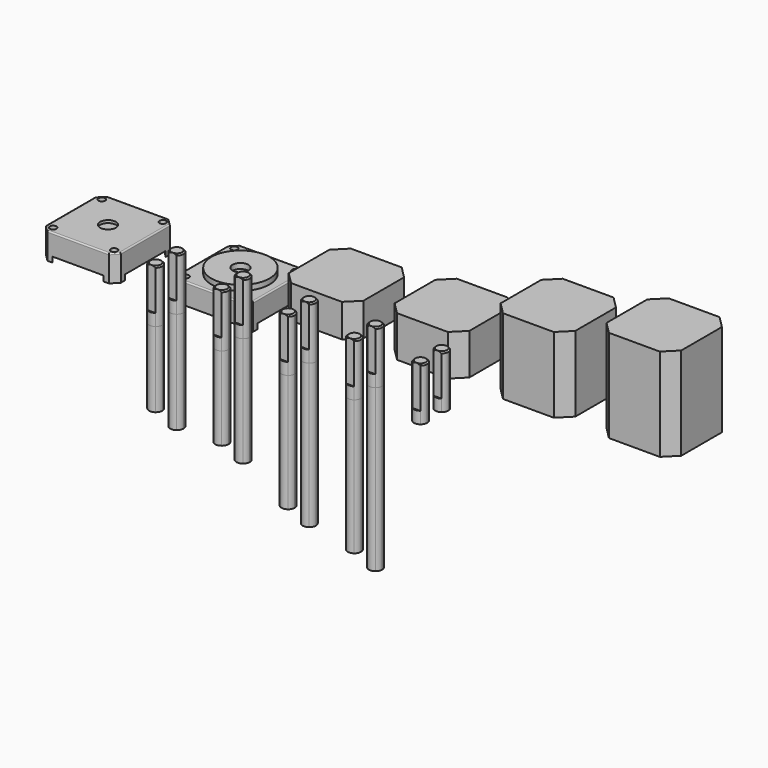
from build123d import *

# Parameters (mm, degrees)
F0_R        = 3
F1_DEPTH    = 8
F0_R_2      = 11
F2_DEPTH    = 2
F3_DEPTH    = 1
F5_DEPTH    = 2
F6_D        = 2.5
F6_DEPTH    = 3
F6_TIP      = 0.7510757738
F6_2_D      = 2.5
F6_2_DEPTH  = 3
F6_2_TIP    = 0.7510757738
F7_DEPTH    = 12.5
F8_DEPTH    = 15.5
F9_DEPTH    = 28.5
F10_DEPTH   = 35
F11_DEPTH   = 20
F13_DEPTH   = 15.5
F14_R       = 0.5
F14_2_R     = 0.5
F15_SIZE    = 0.49999
F15_2_SIZE  = 0.49999
F15_3_SIZE  = 0.49999
F15_4_SIZE  = 0.49999
F15_5_SIZE  = 0.49999
F15_6_SIZE  = 0.49999
F15_7_SIZE  = 0.49999
F15_8_SIZE  = 0.49999
F15_9_SIZE  = 0.49999
F15_10_SIZE = 0.49999
F16_DEPTH   = 28.5
F17_DEPTH   = 38.5
F18_DEPTH   = 31.5
F19_DEPTH   = 41.5
F20_DEPTH   = 44.5
F21_DEPTH   = 54.5
F22_DEPTH   = 51
F23_DEPTH   = 61


# Not quite as in the source:
# - a fillet or chamfer is up to 0.001 mm smaller than in the source, because OpenCascade refuses the exact size
# - a feature names something its author has since deleted; it is built from what else it names


with BuildPart() as f1:
    # F0 (on Top) → F1 (new body)
    with BuildSketch(Plane.XY):
        Polygon((-64.1, 9.6), (-64.1, -9.6), (-59.6, -14.1), (-40.4, -14.1), (-35.9, -9.6), (-35.9, 9.6), (-40.4, 14.1), (-59.6, 14.1), align=None)
        with Locations((-50, 0)):
            Circle(F0_R, mode=Mode.SUBTRACT)
        Polygon((-38.4, 14.1), (-40.4, 14.1), (-35.9, 9.6), (-35.9, 11.6), align=None)
        Polygon((-64.1, 11.6), (-64.1, 9.6), (-59.6, 14.1), (-61.6, 14.1), align=None)
        Polygon((-64.1, -9.6), (-64.1, -11.6), (-61.6, -14.1), (-59.6, -14.1), align=None)
        Polygon((-35.9, -9.6), (-40.4, -14.1), (-38.4, -14.1), (-35.9, -11.6), align=None)
        with Locations((-50, 0)):
            Circle(F0_R)
    extrude(amount=-F1_DEPTH)

    # F0 (on Top) → F3 (cut)
    with BuildSketch(Plane.XY):
        with Locations((-50, 0)):
            Circle(F0_R)
    extrude(amount=-F3_DEPTH, mode=Mode.SUBTRACT)

    # F4 (on face) → F5 (join)
    with BuildSketch(Plane(origin=(0, 0, -8), x_dir=(1, 0, 0), z_dir=(0, 0, -1))):
        Polygon((-35.9, -9.6), (-40.4, -14.1), (-38.4, -14.1), (-35.9, -11.6), align=None)
        Polygon((-61.6, -14.1), (-59.6, -14.1), (-64.1, -9.6), (-64.1, -11.6), align=None)
        Polygon((-64.1, 9.6), (-59.6, 14.1), (-61.6, 14.1), (-64.1, 11.6), align=None)
        Polygon((-35.9, 9.6), (-35.9, 11.6), (-38.4, 14.1), (-40.4, 14.1), align=None)
    extrude(amount=F5_DEPTH)

    # F6
    with Locations(Plane.XY):
        with Locations((-11.5, -11.5), (11.5, -11.5), (11.5, 11.5), (-11.5, 11.5), (-38.5, -11.5), (-38.5, 11.5), (-61.5, 11.5), (-61.5, -11.5)):
            Hole(F6_D / 2, depth=F6_DEPTH)
            with Locations((0, 0, -(F6_DEPTH + F6_TIP / 2))):  # 118° drill point
                Cone(0, F6_D / 2, F6_TIP, mode=Mode.SUBTRACT)

    # F14
    f14_edges = [f1.edges().sort_by_distance(p)[0] for p in [
        (-35.9, 0, 0),
        (-37.15, -12.85, 0),
        (-62.85, -12.85, 0),
        (-64.1, 0, 0),
        (-50, -14.1, 0),
        (-50, 14.1, 0),
        (-37.15, 12.85, 0),
        (-62.85, 12.85, 0),
    ]]
    fillet(f14_edges, radius=F14_R)


with BuildPart() as f1b:
    # F0 (on Top) → F1, piece 2 (new body)
    with BuildSketch(Plane.XY):
        Polygon((-9.6, -14.1), (9.6, -14.1), (14.1, -9.6), (14.1, 9.6), (9.6, 14.1), (-9.6, 14.1), (-14.1, 9.6), (-14.1, -9.6), align=None)
        Circle(F0_R_2, mode=Mode.SUBTRACT)
        Circle(F0_R_2)
        Circle(F0_R, mode=Mode.SUBTRACT)
        Polygon((-11.6, -14.1), (-9.6, -14.1), (-14.1, -9.6), (-14.1, -11.6), align=None)
        Polygon((-14.1, 11.6), (-14.1, 9.6), (-9.6, 14.1), (-11.6, 14.1), align=None)
        Polygon((9.6, 14.1), (14.1, 9.6), (14.1, 11.6), (11.6, 14.1), align=None)
        Polygon((9.6, -14.1), (11.6, -14.1), (14.1, -11.6), (14.1, -9.6), align=None)
        Circle(F0_R)
    extrude(amount=-F1_DEPTH)

    # F0 (on Top) → F2 (join)
    with BuildSketch(Plane.XY):
        Circle(F0_R_2)
        Circle(F0_R, mode=Mode.SUBTRACT)
    extrude(amount=F2_DEPTH)

    # F4 (on face) → F5, piece 2 (join)
    with BuildSketch(Plane(origin=(0, 0, -8), x_dir=(1, 0, 0), z_dir=(0, 0, -1))):
        Polygon((-11.6, -14.1), (-9.6, -14.1), (-14.1, -9.6), (-14.1, -11.6), align=None)
        Polygon((14.1, -9.6), (9.6, -14.1), (11.6, -14.1), (14.1, -11.6), align=None)
        Polygon((9.6, 14.1), (14.1, 9.6), (14.1, 11.6), (11.6, 14.1), align=None)
        Polygon((-14.1, 11.6), (-14.1, 9.6), (-9.6, 14.1), (-11.6, 14.1), align=None)
    extrude(amount=F5_DEPTH)

    # F6#2
    with Locations(Plane.XY):
        with Locations((-11.5, -11.5), (11.5, -11.5), (11.5, 11.5), (-11.5, 11.5), (-38.5, -11.5), (-38.5, 11.5), (-61.5, 11.5), (-61.5, -11.5)):
            Hole(F6_2_D / 2, depth=F6_2_DEPTH)
            with Locations((0, 0, -(F6_2_DEPTH + F6_2_TIP / 2))):  # 118° drill point
                Cone(0, F6_2_D / 2, F6_2_TIP, mode=Mode.SUBTRACT)

    # F14#2
    f14_2_edges = [f1b.edges().sort_by_distance(p)[0] for p in [
        (-14.1, 0, 0),
        (-12.85, -12.85, 0),
        (0, -14.1, 0),
        (12.85, -12.85, 0),
        (14.1, 0, 0),
        (12.85, 12.85, 0),
        (0, 14.1, 0),
        (-12.85, 12.85, 0),
    ]]
    fillet(f14_2_edges, radius=F14_2_R)


with BuildPart() as f7:
    # F0 (on Top) → F7 (new body)
    with BuildSketch(Plane.XY):
        Polygon((30.4, -14.1), (49.6, -14.1), (54.1, -9.6), (54.1, 9.6), (49.6, 14.1), (30.4, 14.1), (25.9, 9.6), (25.9, -9.6), align=None)
    extrude(amount=F7_DEPTH)


with BuildPart() as f8:
    # F0 (on Top) → F8 (new body)
    with BuildSketch(Plane.XY):
        Polygon((70.4, -14.1), (89.6, -14.1), (94.1, -9.6), (94.1, 9.6), (89.6, 14.1), (70.4, 14.1), (65.9, 9.6), (65.9, -9.6), align=None)
    extrude(amount=F8_DEPTH)


with BuildPart() as f9:
    # F0 (on Top) → F9 (new body)
    with BuildSketch(Plane.XY):
        Polygon((110.4, -14.1), (129.6, -14.1), (134.1, -9.6), (134.1, 9.6), (129.6, 14.1), (110.4, 14.1), (105.9, 9.6), (105.9, -9.6), align=None)
    extrude(amount=F9_DEPTH)


with BuildPart() as f10:
    # F0 (on Top) → F10 (new body)
    with BuildSketch(Plane.XY):
        Polygon((150.4, -14.1), (169.6, -14.1), (174.1, -9.6), (174.1, 9.6), (169.6, 14.1), (150.4, 14.1), (145.9, 9.6), (145.9, -9.6), align=None)
    extrude(amount=F10_DEPTH)


with BuildPart() as f11:
    # F0 (on Top) → F11 (new body)
    with BuildSketch(Plane.XY):
        with BuildLine():
            Line((1.5, -42), (-1.5, -42))
            ThreePointArc((-1.5, -42), (0, -42.5), (1.5, -42))
        make_face()
        with BuildLine():
            ThreePointArc((1.5, -42), (2.2360679775, -41.1180339887), (2.5, -40))
            ThreePointArc((2.5, -40), (-1.1180339887, -37.7639320225), (-1.5, -42))
            Line((-1.5, -42), (1.5, -42))
        make_face()
    extrude(amount=F11_DEPTH)


with BuildPart() as f11b:
    # F0 (on Top) → F11, piece 2 (new body)
    with BuildSketch(Plane.XY):
        with BuildLine():
            Line((1.5, -32), (-1.5, -32))
            ThreePointArc((-1.5, -32), (0, -32.5), (1.5, -32))
        make_face()
        with BuildLine():
            ThreePointArc((1.5, -32), (2.2360679775, -31.1180339887), (2.5, -30))
            ThreePointArc((2.5, -30), (-1.1180339887, -27.7639320225), (-1.5, -32))
            Line((-1.5, -32), (1.5, -32))
        make_face()
    extrude(amount=F11_DEPTH)


with BuildPart() as f11c:
    # F0 (on Top) → F11, piece 3 (new body)
    with BuildSketch(Plane.XY):
        with BuildLine():
            ThreePointArc((26.5, -42), (27.2360679775, -41.1180339887), (27.5, -40))
            ThreePointArc((27.5, -40), (23.8819660113, -37.7639320225), (23.5, -42))
            Line((23.5, -42), (26.5, -42))
        make_face()
        with BuildLine():
            Line((26.5, -42), (23.5, -42))
            ThreePointArc((23.5, -42), (25, -42.5), (26.5, -42))
        make_face()
    extrude(amount=F11_DEPTH)


with BuildPart() as f11d:
    # F0 (on Top) → F11, piece 4 (new body)
    with BuildSketch(Plane.XY):
        with BuildLine():
            ThreePointArc((26.5, -32), (27.2360679775, -31.1180339887), (27.5, -30))
            ThreePointArc((27.5, -30), (23.8819660113, -27.7639320225), (23.5, -32))
            Line((23.5, -32), (26.5, -32))
        make_face()
        with BuildLine():
            Line((26.5, -32), (23.5, -32))
            ThreePointArc((23.5, -32), (25, -32.5), (26.5, -32))
        make_face()
    extrude(amount=F11_DEPTH)


with BuildPart() as f11e:
    # F0 (on Top) → F11, piece 5 (new body)
    with BuildSketch(Plane.XY):
        with BuildLine():
            ThreePointArc((51.5, -32), (52.2360679775, -31.1180339887), (52.5, -30))
            ThreePointArc((52.5, -30), (48.8819660113, -27.7639320225), (48.5, -32))
            Line((48.5, -32), (51.5, -32))
        make_face()
        with BuildLine():
            Line((51.5, -32), (48.5, -32))
            ThreePointArc((48.5, -32), (50, -32.5), (51.5, -32))
        make_face()
    extrude(amount=F11_DEPTH)


with BuildPart() as f11f:
    # F0 (on Top) → F11, piece 6 (new body)
    with BuildSketch(Plane.XY):
        with BuildLine():
            ThreePointArc((51.5, -42), (52.2360679775, -41.1180339887), (52.5, -40))
            ThreePointArc((52.5, -40), (48.8819660113, -37.7639320225), (48.5, -42))
            Line((48.5, -42), (51.5, -42))
        make_face()
        with BuildLine():
            Line((51.5, -42), (48.5, -42))
            ThreePointArc((48.5, -42), (50, -42.5), (51.5, -42))
        make_face()
    extrude(amount=F11_DEPTH)


with BuildPart() as f11g:
    # F0 (on Top) → F11, piece 7 (new body)
    with BuildSketch(Plane.XY):
        with BuildLine():
            Line((101.5, -32), (98.5, -32))
            ThreePointArc((98.5, -32), (100, -32.5), (101.5, -32))
        make_face()
        with BuildLine():
            ThreePointArc((101.5, -32), (102.2360679775, -31.1180339887), (102.5, -30))
            ThreePointArc((102.5, -30), (98.8819660113, -27.7639320225), (98.5, -32))
            Line((98.5, -32), (101.5, -32))
        make_face()
    extrude(amount=F11_DEPTH)


with BuildPart() as f11h:
    # F0 (on Top) → F11, piece 8 (new body)
    with BuildSketch(Plane.XY):
        with BuildLine():
            ThreePointArc((101.5, -42), (102.2360679775, -41.1180339887), (102.5, -40))
            ThreePointArc((102.5, -40), (98.8819660113, -37.7639320225), (98.5, -42))
            Line((98.5, -42), (101.5, -42))
        make_face()
        with BuildLine():
            Line((101.5, -42), (98.5, -42))
            ThreePointArc((98.5, -42), (100, -42.5), (101.5, -42))
        make_face()
    extrude(amount=F11_DEPTH)


with BuildPart() as f11i:
    # F0 (on Top) → F11, piece 9 (new body)
    with BuildSketch(Plane.XY):
        with BuildLine():
            ThreePointArc((76.5, -32), (77.2360679775, -31.1180339887), (77.5, -30))
            ThreePointArc((77.5, -30), (73.8819660113, -27.7639320225), (73.5, -32))
            Line((73.5, -32), (76.5, -32))
        make_face()
        with BuildLine():
            Line((76.5, -32), (73.5, -32))
            ThreePointArc((73.5, -32), (75, -32.5), (76.5, -32))
        make_face()
    extrude(amount=F11_DEPTH)


with BuildPart() as f11j:
    # F0 (on Top) → F11, piece 10 (new body)
    with BuildSketch(Plane.XY):
        with BuildLine():
            ThreePointArc((76.5, -42), (77.2360679775, -41.1180339887), (77.5, -40))
            ThreePointArc((77.5, -40), (73.8819660113, -37.7639320225), (73.5, -42))
            Line((73.5, -42), (76.5, -42))
        make_face()
        with BuildLine():
            Line((76.5, -42), (73.5, -42))
            ThreePointArc((73.5, -42), (75, -42.5), (76.5, -42))
        make_face()
    extrude(amount=F11_DEPTH)


with BuildPart() as f13_tool:
    # F12 (on face) → F13 (new body)
    with BuildSketch(Plane.XY.offset(20)):
        with BuildLine():
            ThreePointArc((98.5, -32), (100, -32.5), (101.5, -32))
            Line((101.5, -32), (98.5, -32))
        make_face()
        with BuildLine():
            ThreePointArc((98.5, -42), (100, -42.5), (101.5, -42))
            Line((101.5, -42), (98.5, -42))
        make_face()
        with BuildLine():
            ThreePointArc((73.5, -42), (75, -42.5), (76.5, -42))
            Line((76.5, -42), (73.5, -42))
        make_face()
        with BuildLine():
            ThreePointArc((73.5, -32), (75, -32.5), (76.5, -32))
            Line((76.5, -32), (73.5, -32))
        make_face()
        with BuildLine():
            ThreePointArc((48.5, -32), (50, -32.5), (51.5, -32))
            Line((51.5, -32), (48.5, -32))
        make_face()
        with BuildLine():
            ThreePointArc((48.5, -42), (50, -42.5), (51.5, -42))
            Line((51.5, -42), (48.5, -42))
        make_face()
        with BuildLine():
            ThreePointArc((23.5, -32), (25, -32.5), (26.5, -32))
            Line((26.5, -32), (23.5, -32))
        make_face()
        with BuildLine():
            ThreePointArc((23.5, -42), (25, -42.5), (26.5, -42))
            Line((26.5, -42), (23.5, -42))
        make_face()
        with BuildLine():
            ThreePointArc((-1.5, -32), (0, -32.5), (1.5, -32))
            Line((1.5, -32), (-1.5, -32))
        make_face()
        with BuildLine():
            ThreePointArc((-1.5, -42), (0, -42.5), (1.5, -42))
            Line((1.5, -42), (-1.5, -42))
        make_face()
    extrude(amount=-F13_DEPTH)


with BuildPart() as f11_1:
    add(f11.part)

    # F13: cut by f13_tool
    add(f13_tool.part, mode=Mode.SUBTRACT)

    # F15 (size 0.5 in the source; OpenCascade refuses exactly that, so slightly less here)
    f15_edges = [f11_1.edges().sort_by_distance(p)[0] for p in [
        (0, -37.5, 20),
    ]]
    chamfer(f15_edges, length=F15_SIZE)

    # F16 (add): a face of the model
    f16_faces = [f11_1.faces().sort_by_distance(p)[0] for p in [
        (0, -40, 0),
    ]]
    extrude(f16_faces, amount=F16_DEPTH)


with BuildPart() as f11b_1:
    add(f11b.part)

    # F13: cut by f13_tool
    add(f13_tool.part, mode=Mode.SUBTRACT)

    # F15#2 (size 0.5 in the source; OpenCascade refuses exactly that, so slightly less here)
    f15_2_edges = [f11b_1.edges().sort_by_distance(p)[0] for p in [
        (0, -27.5, 20),
    ]]
    chamfer(f15_2_edges, length=F15_2_SIZE)

    # F17 (add): a face of the model
    f17_faces = [f11b_1.faces().sort_by_distance(p)[0] for p in [
        (0, -30, 0),
    ]]
    extrude(f17_faces, amount=F17_DEPTH)


with BuildPart() as f11c_1:
    add(f11c.part)

    # F13: cut by f13_tool
    add(f13_tool.part, mode=Mode.SUBTRACT)

    # F15#4 (size 0.5 in the source; OpenCascade refuses exactly that, so slightly less here)
    f15_4_edges = [f11c_1.edges().sort_by_distance(p)[0] for p in [
        (23.881966, -37.763932, 20),
    ]]
    chamfer(f15_4_edges, length=F15_4_SIZE)

    # F18 (add): a face of the model
    f18_faces = [f11c_1.faces().sort_by_distance(p)[0] for p in [
        (25, -40, 0),
    ]]
    extrude(f18_faces, amount=F18_DEPTH)


with BuildPart() as f11d_1:
    add(f11d.part)

    # F13: cut by f13_tool
    add(f13_tool.part, mode=Mode.SUBTRACT)

    # F15#3 (size 0.5 in the source; OpenCascade refuses exactly that, so slightly less here)
    f15_3_edges = [f11d_1.edges().sort_by_distance(p)[0] for p in [
        (23.881966, -27.763932, 20),
    ]]
    chamfer(f15_3_edges, length=F15_3_SIZE)

    # F19 (add): a face of the model
    f19_faces = [f11d_1.faces().sort_by_distance(p)[0] for p in [
        (25, -30, 0),
    ]]
    extrude(f19_faces, amount=F19_DEPTH)


with BuildPart() as f11e_1:
    add(f11e.part)

    # F13: cut by f13_tool
    add(f13_tool.part, mode=Mode.SUBTRACT)

    # F15#6 (size 0.5 in the source; OpenCascade refuses exactly that, so slightly less here)
    f15_6_edges = [f11e_1.edges().sort_by_distance(p)[0] for p in [
        (48.881966, -27.763932, 20),
    ]]
    chamfer(f15_6_edges, length=F15_6_SIZE)

    # F21 (add): a face of the model
    f21_faces = [f11e_1.faces().sort_by_distance(p)[0] for p in [
        (50, -30, 0),
    ]]
    extrude(f21_faces, amount=F21_DEPTH)


with BuildPart() as f11f_1:
    add(f11f.part)

    # F13: cut by f13_tool
    add(f13_tool.part, mode=Mode.SUBTRACT)

    # F15#5 (size 0.5 in the source; OpenCascade refuses exactly that, so slightly less here)
    f15_5_edges = [f11f_1.edges().sort_by_distance(p)[0] for p in [
        (48.881966, -37.763932, 20),
    ]]
    chamfer(f15_5_edges, length=F15_5_SIZE)

    # F20 (add): a face of the model
    f20_faces = [f11f_1.faces().sort_by_distance(p)[0] for p in [
        (50, -40, 0),
    ]]
    extrude(f20_faces, amount=F20_DEPTH)


with BuildPart() as f11g_1:
    add(f11g.part)

    # F13: cut by f13_tool
    add(f13_tool.part, mode=Mode.SUBTRACT)

    # F15#10 (size 0.5 in the source; OpenCascade refuses exactly that, so slightly less here)
    f15_10_edges = [f11g_1.edges().sort_by_distance(p)[0] for p in [
        (100, -27.5, 20),
    ]]
    chamfer(f15_10_edges, length=F15_10_SIZE)


with BuildPart() as f11h_1:
    add(f11h.part)

    # F13: cut by f13_tool
    add(f13_tool.part, mode=Mode.SUBTRACT)

    # F15#9 (size 0.5 in the source; OpenCascade refuses exactly that, so slightly less here)
    f15_9_edges = [f11h_1.edges().sort_by_distance(p)[0] for p in [
        (98.881966, -37.763932, 20),
    ]]
    chamfer(f15_9_edges, length=F15_9_SIZE)


with BuildPart() as f11i_1:
    add(f11i.part)

    # F13: cut by f13_tool
    add(f13_tool.part, mode=Mode.SUBTRACT)

    # F15#7 (size 0.5 in the source; OpenCascade refuses exactly that, so slightly less here)
    f15_7_edges = [f11i_1.edges().sort_by_distance(p)[0] for p in [
        (73.881966, -27.763932, 20),
    ]]
    chamfer(f15_7_edges, length=F15_7_SIZE)

    # F23 (add): a face of the model
    f23_faces = [f11i_1.faces().sort_by_distance(p)[0] for p in [
        (75, -30, 0),
    ]]
    extrude(f23_faces, amount=F23_DEPTH)


with BuildPart() as f11j_1:
    add(f11j.part)

    # F13: cut by f13_tool
    add(f13_tool.part, mode=Mode.SUBTRACT)

    # F15#8 (size 0.5 in the source; OpenCascade refuses exactly that, so slightly less here)
    f15_8_edges = [f11j_1.edges().sort_by_distance(p)[0] for p in [
        (73.881966, -37.763932, 20),
    ]]
    chamfer(f15_8_edges, length=F15_8_SIZE)

    # F22 (add): a face of the model
    f22_faces = [f11j_1.faces().sort_by_distance(p)[0] for p in [
        (75, -40, 0),
    ]]
    extrude(f22_faces, amount=F22_DEPTH)


solid = Compound([f1.part, f1b.part, f7.part, f8.part, f9.part, f10.part, f11_1.part, f11b_1.part, f11c_1.part, f11d_1.part, f11e_1.part, f11f_1.part, f11g_1.part, f11h_1.part, f11i_1.part, f11j_1.part])
